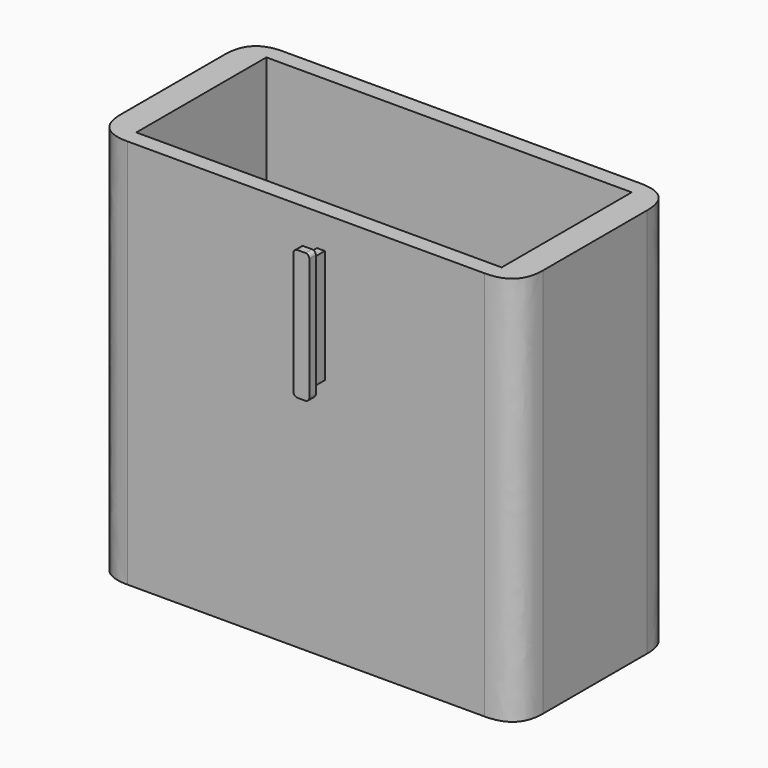
from build123d import *

# Parameters (mm, degrees)
F0_W         = 82.5909674168
F0_H         = 76.3229075819
F1_DEPTH     = 25.4
F3_DEPTH     = 12.7
F4_W         = 71.4602097869
F4_H         = 31.8052172609
F5_DEPTH     = 63.5
F6_W         = 1.5378370881
F6_H         = 22.2577918321
F7_DEPTH     = 3.175
F9_DEPTH     = 1.5875
F10_R        = 0.762
F11_T1_DEPTH = 108.0729075819


# Not quite as in the source:
# - a fillet or chamfer that OpenCascade refuses, or shapes differently, is made with other operations: its cross-section is extruded or revolved along the edge and cut away or added
# - a length typed as a fraction of an inch, garbled in the dataset ("3 / 203.2 mm" for 3/8 in), is restored


with BuildPart() as f1:
    # F0 (on Front) → F1 (new body)
    with BuildSketch(Plane.XZ):
        with Locations((8.6646787822, 7.5585497543)):
            Rectangle(F0_W, F0_H)
    extrude(amount=F1_DEPTH)

    # F3 (add): a face of the model
    f3_faces = [f1.faces().sort_by_distance(p)[0] for p in [
        (8.6646787822, -25.4, 7.5585497543),
    ]]
    extrude(f3_faces, amount=F3_DEPTH)

    # F4 (on face) → F5 (cut)
    with BuildSketch(Plane.XY.offset(45.7200035453)):
        with Locations((8.6646787822, -19.05)):
            Rectangle(F4_W, F4_H)
    extrude(amount=-F5_DEPTH, mode=Mode.SUBTRACT)

    # F6 (on face) → F7 (join)
    with BuildSketch(Plane.XZ.offset(38.1)):
        with Locations((11.5634491667, 28.2745240256)):
            Rectangle(F6_W, F6_H)
    extrude(amount=F7_DEPTH)

    # F11: fillet of radius 6.35 on 4 edges, made by hand

    # F11_s2 → F11_t1 (cut)
    with BuildSketch(Plane.XY.offset(-46.4779040366)):
        with BuildLine():
            add(Edge.make_bspline(
                [(-26.2808049262, 0), (-32.6308049262, 0), (-32.6308049262, -6.35)],
                knots=[0, 0, 0, 1, 1, 1], degree=2, weights=[1, 1, 1]))
            Line((-32.6308049262, -6.35), (-32.6308049262, 0))
            Line((-32.6308049262, 0), (-26.2808049262, 0))
        make_face()
        with BuildLine():
            add(Edge.make_bspline(
                [(-26.2808049262, -38.1), (-32.6308049262, -38.1), (-32.6308049262, -31.75)],
                knots=[0, 0, 0, 1, 1, 1], degree=2, weights=[1, 1, 1]))
            Line((-32.6308049262, -31.75), (-32.6308049262, -38.1))
            Line((-32.6308049262, -38.1), (-26.2808049262, -38.1))
        make_face()
        with BuildLine():
            add(Edge.make_bspline(
                [(49.9601624906, -6.35), (49.9601624906, 0), (43.6101624906, 0)],
                knots=[0, 0, 0, 1, 1, 1], degree=2, weights=[1, 1, 1]))
            Line((43.6101624906, 0), (49.9601624906, 0))
            Line((49.9601624906, 0), (49.9601624906, -6.35))
        make_face()
        with BuildLine():
            add(Edge.make_bspline(
                [(49.9601624906, -31.75), (49.9601624906, -38.1), (43.6101624906, -38.1)],
                knots=[0, 0, 0, 1, 1, 1], degree=2, weights=[1, 1, 1]))
            Line((43.6101624906, -38.1), (49.9601624906, -38.1))
            Line((49.9601624906, -38.1), (49.9601624906, -31.75))
        make_face()
    extrude(amount=F11_T1_DEPTH, mode=Mode.SUBTRACT)


with BuildPart() as f9:
    # F8 (on face) → F9 (new body)
    with BuildSketch(Plane.XZ.offset(41.275)):
        Polygon((10.0171929225, 40.99727422), (10.0171929225, 39.4034199417), (10.0171929225, 17.1456281096), (10.0171929225, 15.5517738312), (13.1097054109, 15.5517738312), (13.1097054109, 17.1456281096), (13.1097054109, 39.4034199417), (13.1097054109, 40.99727422), align=None)
    extrude(amount=F9_DEPTH)

    # F10
    f10_edges = [f9.edges().sort_by_distance(p)[0] for p in [
        (13.109705, -42.06875, 40.997274),
        (10.017193, -42.06875, 40.997274),
        (13.109705, -42.06875, 15.551774),
        (10.017193, -42.06875, 15.551774),
    ]]
    fillet(f10_edges, radius=F10_R)


solid = Compound([f1.part, f9.part])
